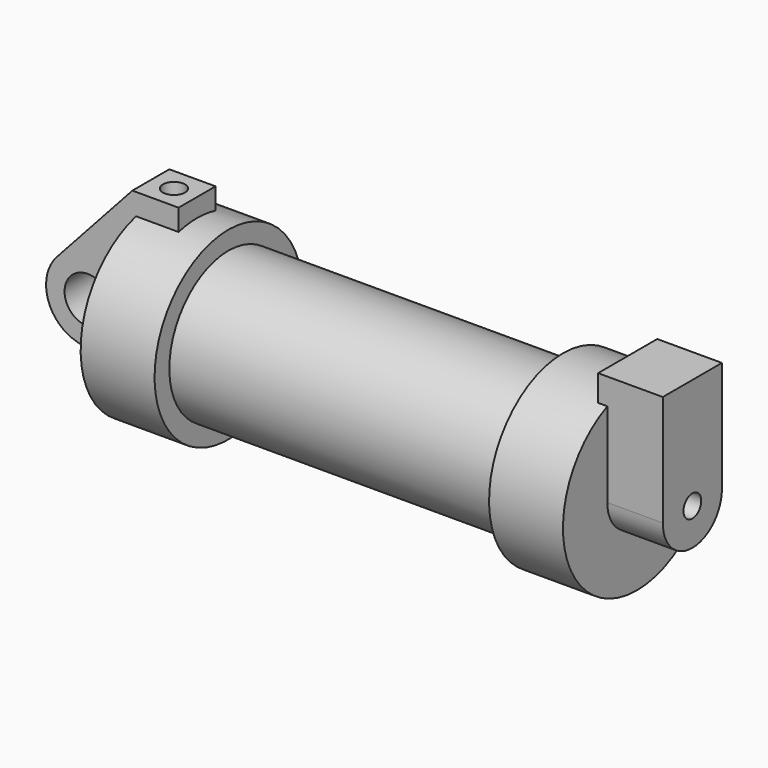
from build123d import *

# Parameters (mm, degrees)
F0_W      = 5.842
F0_H      = 12.7
F0_R      = 3.175
F2_DEPTH  = 3.175
F5_DEPTH  = 1.27
F4_R      = 1.524
F6_DEPTH  = 7.62
F10_R     = 1.524
F11_DEPTH = 17.78


# Not quite as in the source:
# - a feature of the source that left no trace in its solid (it failed there, or was rolled back) is left out


with BuildPart() as f1:
    # F0 (on Front) → F1 (revolve)
    with BuildSketch(Plane.XZ):
        Polygon((5.842, 12.7), (5.842, 0), (66.294, 0), (66.294, 12.7), (56.134, 12.7), (56.134, 10.16), (10.16, 10.16), (10.16, 12.7), align=None)
        with Locations((2.921, 6.35)):
            Rectangle(F0_W, F0_H)
    revolve(axis=Axis((33.147, 0, 0), (-1, 0, 0)))

    # F0 (on Front) → F2 (join, symmetric)
    with BuildSketch(Plane.XZ):
        with BuildLine():
            Line((5.842, 0), (0, 0))
            Line((0, 0), (-0.9398, 0))
            ThreePointArc((-0.9398, 0), (-3.1957909266, -4.5493385486), (-8.1826630726, -5.5069827884))
            Line((-8.1826630726, -5.5069827884), (5.842, -9.398))
            Line((5.842, -9.398), (5.842, 0))
        make_face()
        with BuildLine():
            Line((-0.9398, 0), (0, 0))
            Line((0, 0), (0, 12.7))
            Line((0, 12.7), (5.842, 12.7))
            Line((5.842, 12.7), (5.842, 15.24))
            Line((5.842, 15.24), (-0.508, 15.24))
            Line((-0.508, 15.24), (-10.8806298187, 3.8475430269))
            ThreePointArc((-10.8806298187, 3.8475430269), (-4.5919612295, 5.3297205562), (-0.9398, 0))
        make_face()
        with BuildLine():
            ThreePointArc((-8.1826630726, -5.5069827884), (-3.1957909266, -4.5493385486), (-0.9398, 0))
            ThreePointArc((-0.9398, 0), (-4.5919612295, 5.3297205562), (-10.8806298187, 3.8475430269))
            ThreePointArc((-10.8806298187, 3.8475430269), (-12.1459778134, -1.5837270034), (-8.1826630726, -5.5069827884))
        make_face()
        with Locations((-6.6548, 0)):
            Circle(F0_R, mode=Mode.SUBTRACT)
        with Locations((2.921, 6.35)):
            Rectangle(F0_W, F0_H)
    extrude(amount=F2_DEPTH, both=True)

    # F3: union 

    # F4 (on face) → F5 (join)
    with BuildSketch(Plane.YZ.offset(66.294)):
        with BuildLine():
            ThreePointArc((-5.08, 11.6397422652), (0, 12.7), (5.08, 11.6397422652))
            Line((5.08, 11.6397422652), (5.08, 15.24))
            Line((5.08, 15.24), (-5.08, 15.24))
            Line((-5.08, 15.24), (-5.08, 11.6397422652))
        make_face()
    extrude(amount=-F5_DEPTH)

    # F4 (on face) → F6 (join)
    with BuildSketch(Plane.YZ.offset(66.294)):
        with BuildLine():
            Line((5.08, 0), (5.08, 11.6397422652))
            ThreePointArc((5.08, 11.6397422652), (0, 12.7), (-5.08, 11.6397422652))
            Line((-5.08, 11.6397422652), (-5.08, 0))
            ThreePointArc((-5.08, 0), (0, 5.08), (5.08, 0))
        make_face()
        with BuildLine():
            ThreePointArc((-5.08, 11.6397422652), (0, 12.7), (5.08, 11.6397422652))
            Line((5.08, 11.6397422652), (5.08, 15.24))
            Line((5.08, 15.24), (-5.08, 15.24))
            Line((-5.08, 15.24), (-5.08, 11.6397422652))
        make_face()
        with BuildLine():
            ThreePointArc((-5.08, 0), (0, -5.08), (5.08, 0))
            ThreePointArc((5.08, 0), (0, 5.08), (-5.08, 0))
        make_face()
        Circle(F4_R, mode=Mode.SUBTRACT)
    extrude(amount=F6_DEPTH)

    # F7: union 

    # F10 (on face) → F11 (cut)
    with BuildSketch(Plane.XY.offset(15.24)):
        with Locations((2.667, 0)):
            Circle(F10_R)
    extrude(amount=-F11_DEPTH, mode=Mode.SUBTRACT)


solid = f1.part
